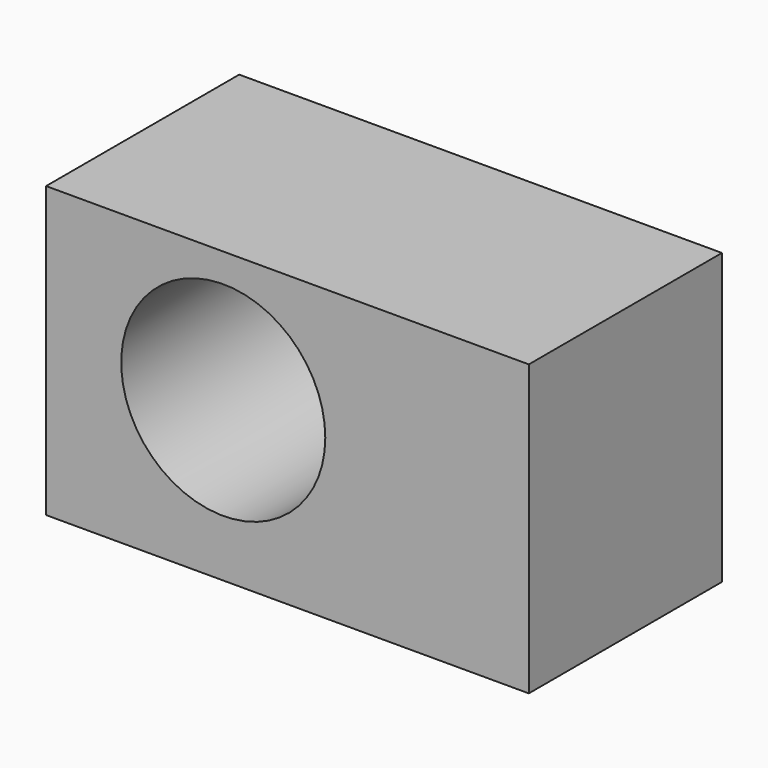
from build123d import *

# Parameters (mm, degrees)
F0_W     = 50
F0_H     = 30
F1_DEPTH = 25
F2_R     = 10.5679387912
F3_DEPTH = 25


# Not quite as in the source:
# - a feature of the source that left no trace in its solid (it failed there, or was rolled back) is left out


with BuildPart() as f1:
    # F0 (on Front) → F1 (new body)
    with BuildSketch(Plane.XZ):
        with Locations((1.7205976233, 19.2674261052)):
            Rectangle(F0_W, F0_H)
    extrude(amount=F1_DEPTH)

    # F2 (on face) → F3 (cut)
    with BuildSketch(Plane.XZ.offset(25)):
        with Locations((-4.9288761802, 20.7236856222)):
            Circle(F2_R)
    extrude(amount=-F3_DEPTH, mode=Mode.SUBTRACT)


solid = f1.part
